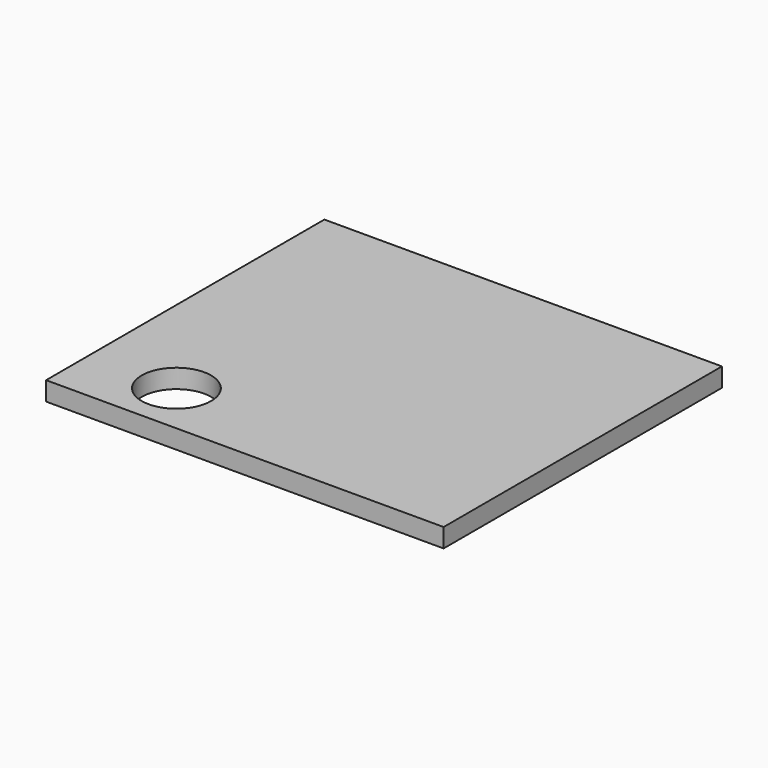
from build123d import *

# Parameters (mm, degrees)
F0_R     = 34.9136260122
F1_DEPTH = 19
F2_DEPTH = 543
F3_DEPTH = 543


# Not quite as in the source:
# - an extrude ends at something that could not be found from the text; its depth is read off the source's solid


with BuildPart() as f1:
    # F0 (on Top) → F1 (new body)
    with BuildSketch(Plane.XY):
        with BuildLine():
            Line((200, 110.9662795378), (200, 175))
            Line((200, 175), (141.3804350425, 175))
            add(Edge.make_bspline(
                [(141.3804350425, 175), (156.8649910086, 175), (190.60117535, 168.7984586395), (200, 130.1435418358), (200, 110.9662795378)],
                knots=[0, 0, 0, 0, 0.4762392851, 1, 1, 1, 1], degree=3))
        make_face()
        with BuildLine():
            add(Edge.make_bspline(
                [(141.3804350425, 175), (156.8649910086, 175), (190.60117535, 168.7984586395), (200, 130.1435418358), (200, 110.9662795378)],
                knots=[0, 0, 0, 0, 0.4762392851, 1, 1, 1, 1], degree=3))
            Line((141.3804350425, 175), (-137.7466996101, 175))
            add(Edge.make_bspline(
                [(-200, 108.9276008911), (-200, 127.4557680251), (-189.1867570844, 163.9441482544), (-156.7886150254, 175), (-137.7466996101, 175)],
                knots=[0, 0, 0, 0, 0.5072026371, 1, 1, 1, 1], degree=3))
            Line((-200, 108.9276008911), (-200, -122.5906014442))
            add(Edge.make_bspline(
                [(-147.5979983807, -175), (-157.9488683475, -174.1189344774), (-192.8861581663, -165.8033781762), (-198.1868907749, -133.2250279634), (-200, -122.5906014442)],
                knots=[0, 0, 0, 0, 0.5043810007, 1, 1, 1, 1], degree=3))
            Line((-147.5979983807, -175), (130.1678889743, -175))
            add(Edge.make_bspline(
                [(200, -116.7001660973), (200, -125.782076666), (189.6771600262, -168.0094712369), (144.6769061507, -175), (130.1678889743, -175)],
                knots=[0, 0, 0, 0, 0.4745951866, 1, 1, 1, 1], degree=3))
            Line((200, -116.7001660973), (200, 110.9662795378))
        make_face()
        with Locations((-111.4690546889, -121.7351463744)):
            Circle(F0_R, mode=Mode.SUBTRACT)
        with BuildLine():
            add(Edge.make_bspline(
                [(-200, 108.9276008911), (-200, 127.4557680251), (-189.1867570844, 163.9441482544), (-156.7886150254, 175), (-137.7466996101, 175)],
                knots=[0, 0, 0, 0, 0.5072026371, 1, 1, 1, 1], degree=3))
            Line((-137.7466996101, 175), (-200, 175))
            Line((-200, 175), (-200, 108.9276008911))
        make_face()
        with BuildLine():
            Line((200, -175), (200, -116.7001660973))
            add(Edge.make_bspline(
                [(200, -116.7001660973), (200, -125.782076666), (189.6771600262, -168.0094712369), (144.6769061507, -175), (130.1678889743, -175)],
                knots=[0, 0, 0, 0, 0.4745951866, 1, 1, 1, 1], degree=3))
            Line((130.1678889743, -175), (200, -175))
        make_face()
        with BuildLine():
            add(Edge.make_bspline(
                [(-147.5979983807, -175), (-157.9488683475, -174.1189344774), (-192.8861581663, -165.8033781762), (-198.1868907749, -133.2250279634), (-200, -122.5906014442)],
                knots=[0, 0, 0, 0, 0.5043810007, 1, 1, 1, 1], degree=3))
            Line((-200, -122.5906014442), (-200, -175))
            Line((-200, -175), (-147.5979983807, -175))
        make_face()
    extrude(amount=F1_DEPTH)

    # F0 (on Top) → F2 (cut, through all)
    with BuildSketch(Plane.XY):
        with Locations((-111.4690546889, -121.7351463744)):
            Circle(F0_R)
    extrude(amount=-F2_DEPTH, mode=Mode.SUBTRACT)

    # F0 (on Top) → F3 (cut, through all)
    with BuildSketch(Plane.XY):
        with BuildLine():
            add(Edge.make_bspline(
                [(-147.5979983807, -175), (-157.9488683475, -174.1189344774), (-192.8861581663, -165.8033781762), (-198.1868907749, -133.2250279634), (-200, -122.5906014442)],
                knots=[0, 0, 0, 0, 0.5043810007, 1, 1, 1, 1], degree=3))
            Line((-200, -122.5906014442), (-200, -175))
            Line((-200, -175), (-147.5979983807, -175))
        make_face()
    extrude(amount=-F3_DEPTH, mode=Mode.SUBTRACT)


solid = f1.part
